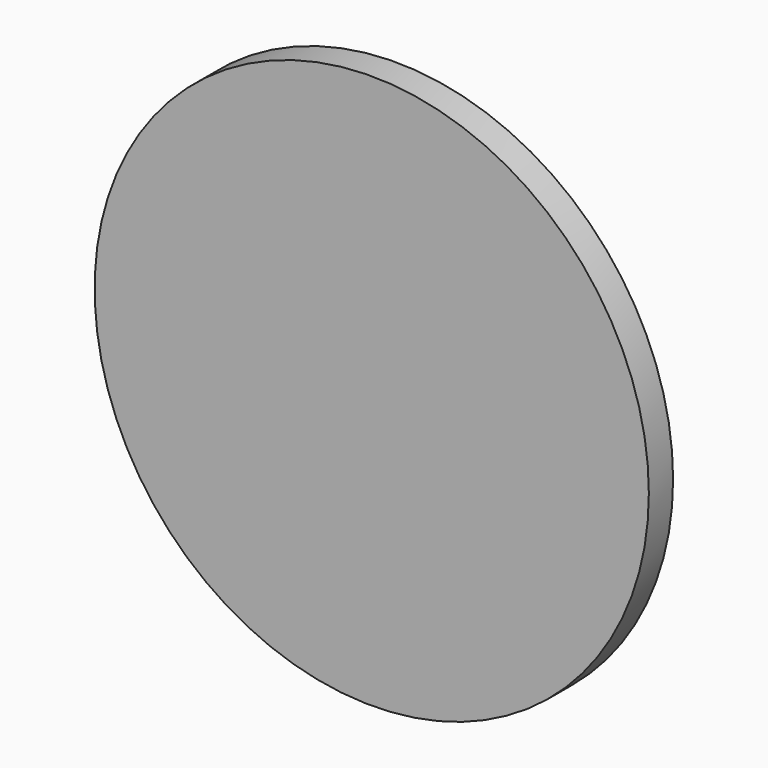
from build123d import *

# Parameters (mm, degrees)
F0_R     = 45.7177259428
F1_DEPTH = 5
F2_R     = 1.5175
F3_DEPTH = 0.3


# Not quite as in the source:
# - a feature names something its author has since deleted; it is built from what else it names


with BuildPart() as f1:
    # F0 (on Front) → F1 (new body)
    with BuildSketch(Plane.XZ):
        with Locations((-222.7153331041, -41.6794866323)):
            Circle(F0_R)
    extrude(amount=F1_DEPTH)

    # F2 (on face) → F3 (join)
    with BuildSketch(Plane.XZ.offset(5)):
        with Locations((-222.7153331041, -41.6794866323)):
            Circle(F2_R)
    extrude(amount=-F3_DEPTH)


solid = f1.part
